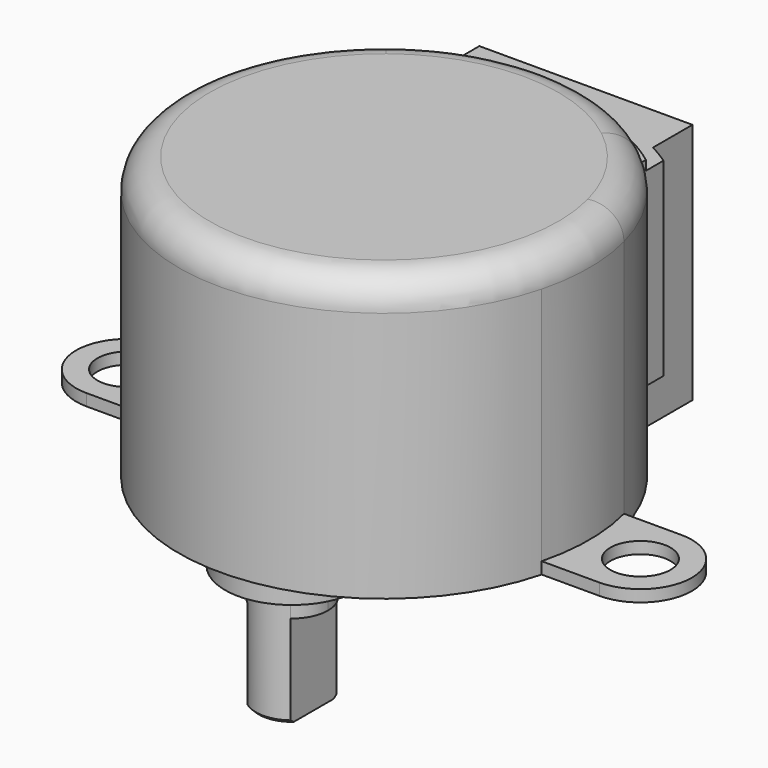
from build123d import *

# Parameters (mm, degrees)
F0_R         = 2.05
F1_DEPTH     = 0.8
F2_DEPTH     = 19.2
F3_R         = 4.55
F4_DEPTH     = 2.1
F5_DEPTH     = 4
F6_DEPTH     = 10.3
F8_W         = 14.5
F8_H         = 16.5
F12_DEPTH    = 13.55
F13_DEPTH    = 0.65
F14_T2_ANGLE = 246.3939611614
F14_T4_ANGLE = 31.9483260065
F14_T6_ANGLE = 44.2717080563
F14_T8_ANGLE = 37.3860047758
F15_SIZE     = 0.2


# Not quite as in the source:
# - a fillet or chamfer that OpenCascade refuses, or shapes differently, is made with other operations: its cross-section is extruded or revolved along the edge and cut away or added


with BuildPart() as f1:
    # F0 (on Top) → F1 (new body)
    with BuildSketch(Plane.XY):
        with BuildLine():
            ThreePointArc((-13.5296202829, -3.5), (-13.975, 0), (-13.5296202829, 3.5))
            Line((-13.5296202829, 3.5), (-17.45, 3.5))
            ThreePointArc((-17.45, 3.5), (-20.95, 0), (-17.45, -3.5))
            Line((-17.45, -3.5), (-13.5296202829, -3.5))
        make_face()
        with Locations((-17.45, 0)):
            Circle(F0_R, mode=Mode.SUBTRACT)
    extrude(amount=F1_DEPTH)



with BuildPart() as f1b:
    # F0 (on Top) → F1, piece 2 (new body)
    with BuildSketch(Plane.XY):
        with BuildLine():
            Line((17.45, 3.5), (13.5296202829, 3.5))
            ThreePointArc((13.5296202829, 3.5), (13.975, 0), (13.5296202829, -3.5))
            Line((13.5296202829, -3.5), (17.45, -3.5))
            ThreePointArc((17.45, -3.5), (20.95, 0), (17.45, 3.5))
        make_face()
        with Locations((17.45, 0)):
            Circle(F0_R, mode=Mode.SUBTRACT)
    extrude(amount=F1_DEPTH)


with BuildPart() as f1_1:
    add(f1.part)

    add(f1b.part)  # F2 merges F1b
    # F0 (on Top) → F2 (join)
    with BuildSketch(Plane.XY):
        with BuildLine():
            ThreePointArc((13.5296202829, -3.5), (13.975, 0), (13.5296202829, 3.5))
            ThreePointArc((13.5296202829, 3.5), (0, 13.975), (-13.5296202829, 3.5))
            ThreePointArc((-13.5296202829, 3.5), (-13.975, 0), (-13.5296202829, -3.5))
            ThreePointArc((-13.5296202829, -3.5), (0, -13.975), (13.5296202829, -3.5))
        make_face()
    extrude(amount=F2_DEPTH)

    # F3 (on Top) → F4 (join)
    with BuildSketch(Plane.XY):
        with Locations((0, -7.825)):
            Circle(F3_R)
        with BuildLine():
            ThreePointArc((1.475, -5.8687599841), (2.1927437151, -6.7321253503), (2.45, -7.825))
            ThreePointArc((2.45, -7.825), (2.1927437151, -8.9178746497), (1.475, -9.7812400159))
            ThreePointArc((1.475, -9.7812400159), (0, -10.275), (-1.475, -9.7812400159))
            ThreePointArc((-1.475, -9.7812400159), (-2.45, -7.825), (-1.475, -5.8687599841))
            ThreePointArc((-1.475, -5.8687599841), (0, -5.375), (1.475, -5.8687599841))
        make_face(mode=Mode.SUBTRACT)
    extrude(amount=-F4_DEPTH)

    # F3 (on Top) → F5 (join)
    with BuildSketch(Plane.XY):
        with BuildLine():
            ThreePointArc((1.475, -9.7812400159), (2.1927437151, -8.9178746497), (2.45, -7.825))
            ThreePointArc((2.45, -7.825), (2.1927437151, -6.7321253503), (1.475, -5.8687599841))
            Line((1.475, -5.8687599841), (1.475, -9.7812400159))
        make_face()
        with BuildLine():
            Line((1.475, -9.7812400159), (1.475, -5.8687599841))
            ThreePointArc((1.475, -5.8687599841), (0, -5.375), (-1.475, -5.8687599841))
            Line((-1.475, -5.8687599841), (-1.475, -9.7812400159))
            ThreePointArc((-1.475, -9.7812400159), (0, -10.275), (1.475, -9.7812400159))
        make_face()
        with BuildLine():
            Line((-1.475, -9.7812400159), (-1.475, -5.8687599841))
            ThreePointArc((-1.475, -5.8687599841), (-2.45, -7.825), (-1.475, -9.7812400159))
        make_face()
    extrude(amount=-F5_DEPTH)

    # F3 (on Top) → F6 (join)
    with BuildSketch(Plane.XY):
        with BuildLine():
            Line((1.475, -9.7812400159), (1.475, -5.8687599841))
            ThreePointArc((1.475, -5.8687599841), (0, -5.375), (-1.475, -5.8687599841))
            Line((-1.475, -5.8687599841), (-1.475, -9.7812400159))
            ThreePointArc((-1.475, -9.7812400159), (0, -10.275), (1.475, -9.7812400159))
        make_face()
    extrude(amount=-F6_DEPTH)

    # F8 (on offset) → F9 (join, up to the next surface of F1)
    with BuildSketch(Plane.XZ.offset(-17.175)):
        with Locations((0, 8.25)):
            Rectangle(F8_W, F8_H)
    extrude(until=Until.NEXT)

    # F11 (on offset) → F12 (join)
    with BuildSketch(Plane.XY.offset(17.15)):
        with BuildLine():
            Line((-8.625, 12.9959083299), (-8.625, 11.5))
            ThreePointArc((-8.625, 11.5), (-7.9506110955, 11.9761599943), (-7.25, 12.4128209928))
            Line((-7.25, 12.4128209928), (-7.25, 13.8205759578))
            ThreePointArc((-7.25, 13.8205759578), (-7.9482026537, 13.4260870893), (-8.625, 12.9959083299))
        make_face()
        with BuildLine():
            ThreePointArc((7.25, 12.4128209928), (7.9506110955, 11.9761599943), (8.625, 11.5))
            Line((8.625, 11.5), (8.625, 12.9959083299))
            ThreePointArc((8.625, 12.9959083299), (7.9482026537, 13.4260870893), (7.25, 13.8205759578))
            Line((7.25, 13.8205759578), (7.25, 12.4128209928))
        make_face()
        with BuildLine():
            Line((8.625, 10.9959083299), (8.625, 11.5))
            ThreePointArc((8.625, 11.5), (7.9506110955, 11.9761599943), (7.25, 12.4128209928))
            ThreePointArc((7.25, 12.4128209928), (4.4752329692, 13.6606337654), (1.5, 14.2965249274))
            Line((1.5, 14.2965249274), (1.5, 13.8942659036))
            ThreePointArc((1.5, 13.8942659036), (5.2658356798, 12.9449449436), (8.625, 10.9959083299))
        make_face()
        with BuildLine():
            Line((-8.625, 11.5), (-8.625, 10.9959083299))
            ThreePointArc((-8.625, 10.9959083299), (-5.2658356798, 12.9449449436), (-1.5, 13.8942659036))
            Line((-1.5, 13.8942659036), (-1.5, 14.2965249274))
            ThreePointArc((-1.5, 14.2965249274), (-4.4752329692, 13.6606337654), (-7.25, 12.4128209928))
            ThreePointArc((-7.25, 12.4128209928), (-7.9506110955, 11.9761599943), (-8.625, 11.5))
        make_face()
    extrude(amount=-F12_DEPTH)

    # F11 (on offset) → F13 (cut, through all)
    with BuildSketch(Plane.XY.offset(17.15)):
        with BuildLine():
            Line((-8.625, 12.9959083299), (-8.625, 11.5))
            ThreePointArc((-8.625, 11.5), (-7.9506110955, 11.9761599943), (-7.25, 12.4128209928))
            Line((-7.25, 12.4128209928), (-7.25, 13.8205759578))
            ThreePointArc((-7.25, 13.8205759578), (-7.9482026537, 13.4260870893), (-8.625, 12.9959083299))
        make_face()
        with BuildLine():
            ThreePointArc((7.25, 12.4128209928), (7.9506110955, 11.9761599943), (8.625, 11.5))
            Line((8.625, 11.5), (8.625, 12.9959083299))
            ThreePointArc((8.625, 12.9959083299), (7.9482026537, 13.4260870893), (7.25, 13.8205759578))
            Line((7.25, 13.8205759578), (7.25, 12.4128209928))
        make_face()
    extrude(amount=-F13_DEPTH, mode=Mode.SUBTRACT)

    # F14: fillet of radius 2.1 on 1 edges, made by hand

    # F14_s1 → F14_t2 (revolve, cut)
    with BuildSketch(Plane(origin=(0, 0, 0), x_dir=(0, 0, 1), z_dir=(-0.2504472272, 0.9681302528, 0))):
        with BuildLine():
            ThreePointArc((17.1, 13.975), (18.5849242405, 13.3599242405), (19.2, 11.875))
            Line((19.2, 11.875), (19.242, 11.875))
            Line((19.242, 11.875), (19.242, 14.017))
            Line((19.242, 14.017), (17.1, 14.017))
            Line((17.1, 14.017), (17.1, 13.975))
        make_face()
    revolve(axis=Axis((0, 0, 19.2), (0, 0, -1)), revolution_arc=F14_T2_ANGLE, mode=Mode.SUBTRACT)

    # F14_s3 → F14_t4 (revolve, cut)
    with BuildSketch(Plane(origin=(0, 0, 0), x_dir=(0, 0, 1), z_dir=(-0.7868271317, -0.617173448, 0))):
        with BuildLine():
            ThreePointArc((17.15, 13.975), (18.6024979201, 13.3427353976), (19.2, 11.8755953225))
            Line((19.2, 11.8755953225), (19.242, 11.8755953225))
            Line((19.242, 11.8755953225), (19.242, 13.975))
            Line((19.242, 13.975), (19.2, 14.017))
            ThreePointArc((19.2, 14.017), (18.175, 14.017), (17.151, 14.0169880936))
            Line((17.151, 14.0169880936), (17.15, 13.975))
        make_face()
    revolve(axis=Axis((0, 0, 19.2), (0, 0, -1)), revolution_arc=F14_T4_ANGLE, mode=Mode.SUBTRACT)

    # F14_s5 → F14_t6 (revolve, cut)
    with BuildSketch(Plane(origin=(0, 0, 0), x_dir=(0, 0, 1), z_dir=(-0.9942229517, -0.1073346275, 0))):
        with BuildLine():
            ThreePointArc((17.15, 13.975), (18.6024979201, 13.3427353976), (19.2, 11.8755953225))
            Line((19.2, 11.8755953225), (19.242, 11.8755953225))
            Line((19.242, 11.8755953225), (19.242, 13.975))
            Line((19.242, 13.975), (19.2, 14.017))
            ThreePointArc((19.2, 14.017), (18.175, 14.017), (17.151, 14.0169880936))
            Line((17.151, 14.0169880936), (17.15, 13.975))
        make_face()
    revolve(axis=Axis((0, 0, 19.2), (0, 0, -1)), revolution_arc=F14_T6_ANGLE, mode=Mode.SUBTRACT)

    # F14_s7 → F14_t8 (revolve, cut)
    with BuildSketch(Plane(origin=(0, 0, 0), x_dir=(0, 0, 1), z_dir=(-0.7868271352, 0.6171734435, 0))):
        with BuildLine():
            ThreePointArc((17.1, 13.975), (18.5849242405, 13.3599242405), (19.2, 11.875))
            Line((19.2, 11.875), (19.242, 11.875))
            Line((19.242, 11.875), (19.242, 14.017))
            Line((19.242, 14.017), (17.1, 14.017))
            Line((17.1, 14.017), (17.1, 13.975))
        make_face()
    revolve(axis=Axis((0, 0, 19.2), (0, 0, -1)), revolution_arc=F14_T8_ANGLE, mode=Mode.SUBTRACT)

    # F15
    f15_edges = [f1_1.edges().sort_by_distance(p)[0] for p in [
        (0, -5.375, -10.3),
        (0, -10.275, -10.3),
    ]]
    chamfer(f15_edges, length=F15_SIZE)


solid = f1_1.part
